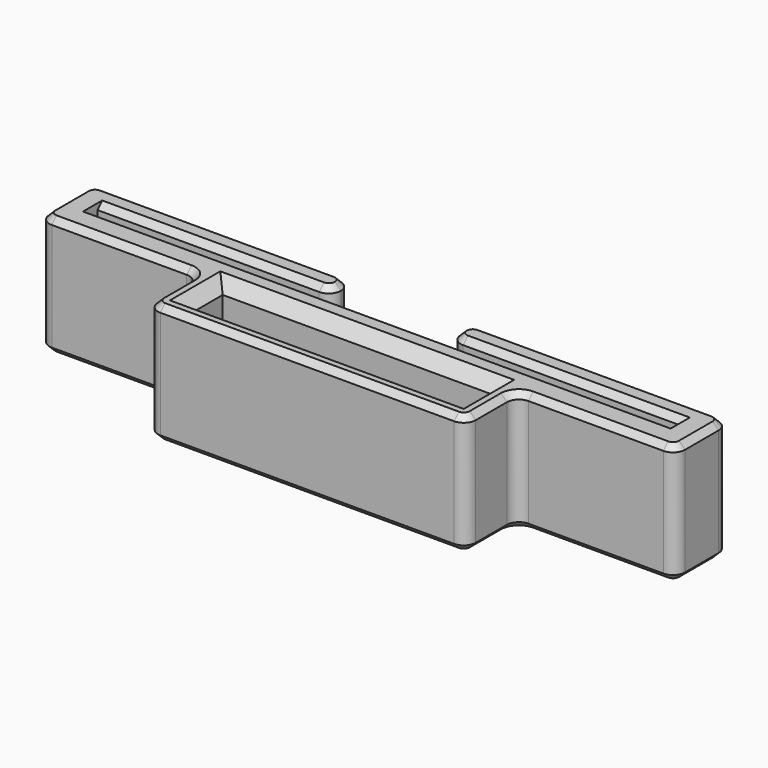
from build123d import *

# Parameters (mm, degrees)
F0_W          = 53
F0_H          = 5.5
F0_W_2        = 49
F0_H_2        = 1.5
F1_DEPTH      = 5
F2_W          = 10
F2_H          = 10
F3_DEPTH      = 2
F5_DEPTH      = 5
F5_DEPTH_BACK = 5
F6_SIZE       = 1
F7_R          = 0.99999
F8_R          = 1
F9_SIZE       = 0.5


# Not quite as in the source:
# - a fillet or chamfer is up to 0.001 mm smaller than in the source, because OpenCascade refuses the exact size


with BuildPart() as f1:
    # F0 (on Top) → F1 (new body, symmetric)
    with BuildSketch(Plane.XY):
        Rectangle(F0_W, F0_H)
        Rectangle(F0_W_2, F0_H_2, mode=Mode.SUBTRACT)
    extrude(amount=F1_DEPTH, both=True)

    # F2 (on face) → F3 (cut, through all)
    with BuildSketch(Plane(origin=(0, 2.75, 0), x_dir=(-1, 0, 0), z_dir=(0, 1, 0))):
        Rectangle(F2_W, F2_H)
    extrude(amount=-F3_DEPTH, mode=Mode.SUBTRACT)

    # F4 (on Top) → F5 (join, two sides)
    with BuildSketch(Plane.XY) as f5_sk:
        Polygon((-13.25, -8), (13.25, -8), (13.25, -2.75), (11.25, -2.75), (11.25, -6), (-11.25, -6), (-11.25, -2.75), (-13.25, -2.75), align=None)
    extrude(amount=F5_DEPTH)
    extrude(f5_sk.sketch, amount=-F5_DEPTH_BACK)

    # F6
    f6_edges = [f1.edges().sort_by_distance(p)[0] for p in [
        (0, -2.75, 5),
        (0, -6, 5),
        (11.25, -4.375, 5),
        (-11.25, -4.375, 5),
    ]]
    chamfer(f6_edges, length=F6_SIZE)

    # F7 (radius 1 in the source; OpenCascade refuses exactly that, so slightly less here)
    f7_edges = [f1.edges().sort_by_distance(p)[0] for p in [
        (-5, 2.75, 0),
        (5, 0.75, 0),
        (5, 2.75, 0),
        (-5, 0.75, 0),
    ]]
    fillet(f7_edges, radius=F7_R)

    # F8
    f8_edges = [f1.edges().sort_by_distance(p)[0] for p in [
        (-13.25, -2.75, 0),
        (-26.5, -2.75, 0),
        (26.5, -2.75, 0),
        (-13.25, -8, 0),
        (26.5, 2.75, 0),
        (13.25, -8, 0),
        (13.25, -2.75, 0),
        (-26.5, 2.75, 0),
    ]]
    fillet(f8_edges, radius=F8_R)

    # F9
    f9_edges = [f1.edges().sort_by_distance(p)[0] for p in [
        (-15.749995, 2.75, -5),
        (-15.749995, 2.75, 5),
    ]]
    chamfer(f9_edges, length=F9_SIZE)


solid = f1.part
